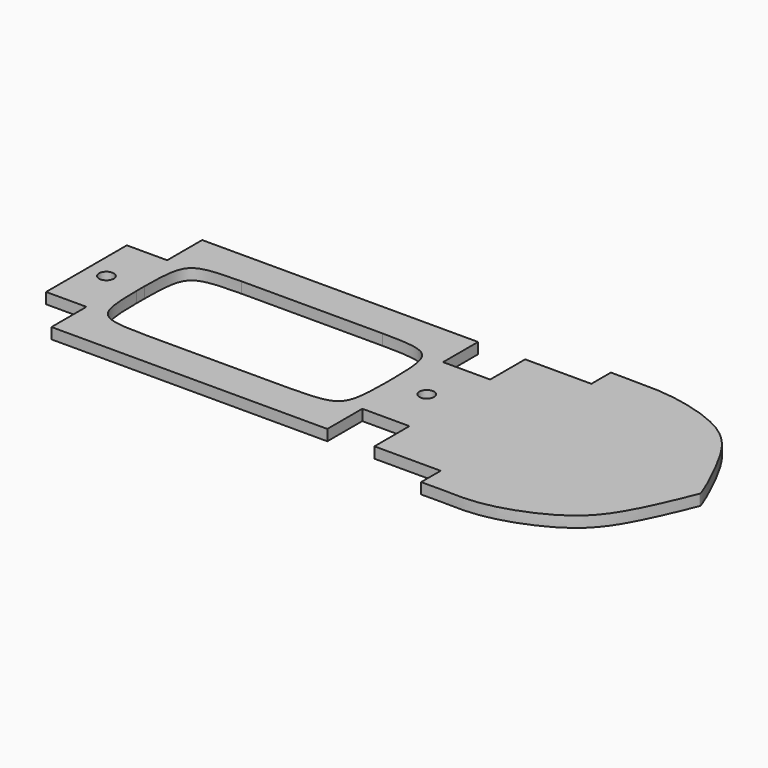
from build123d import *

# Parameters (mm, degrees)
F0_W        = 41.91
F0_H        = 19.05
F0_R        = 1.3890625
F0_W_2      = 52.07
F0_H_2      = 8.255
F0_W_3      = 7.62
F1_DEPTH    = 2.0574
F2_W        = 46.99
F2_H        = 22.225
F3_DEPTH    = 25.4
F4_T1_DEPTH = 2.0574
F6_DEPTH    = 2.0574


# Not quite as in the source:
# - a fillet or chamfer that OpenCascade refuses, or shapes differently, is made with other operations: its cross-section is extruded or revolved along the edge and cut away or added
# - a feature names something its author has since deleted; it is built from what else it names


with BuildPart() as f1:
    # F0 (on Top) → F1 (new body)
    with BuildSketch(Plane.XY):
        with Locations((29.845, 0)):
            Rectangle(F0_W, F0_H)
        with Locations((13.4267662017, 0)):
            Circle(F0_R, mode=Mode.SUBTRACT)
        with Locations((-17.145, -13.6525)):
            Rectangle(F0_W_2, F0_H_2)
        with Locations((-17.145, 0)):
            Rectangle(F0_W_2, F0_H)
        with Locations((-46.99, 0)):
            Rectangle(F0_W_3, F0_H)
        with Locations((-47.0252337983, 0)):
            Circle(F0_R, mode=Mode.SUBTRACT)
        with Locations((-17.145, 13.6525)):
            Rectangle(F0_W_2, F0_H_2)
    extrude(amount=F1_DEPTH)

    # F2 (on face) → F3 (cut)
    with BuildSketch(Plane.XY.offset(2.0574)):
        with Locations((-17.0991587498, 0)):
            Rectangle(F2_W, F2_H)
    extrude(amount=-F3_DEPTH, mode=Mode.SUBTRACT)

    # F4: fillet of radius 10.16 on 4 edges, made by hand

    # F4_s2 → F4_t1 (join)
    with BuildSketch(Plane.XY):
        with BuildLine():
            add(Edge.make_bspline(
                [(6.3958412502, 0.9525), (6.3958412502, 11.1125), (-3.7641587498, 11.1125)],
                knots=[0, 0, 0, 1, 1, 1], degree=2, weights=[1, 2.3333333333, 1]))
            Line((-3.7641587498, 11.1125), (6.3958412502, 11.1125))
            Line((6.3958412502, 11.1125), (6.3958412502, 0.9525))
        make_face()
        with BuildLine():
            add(Edge.make_bspline(
                [(-30.4341587498, 11.1125), (-40.5941587498, 11.1125), (-40.5941587498, 0.9525)],
                knots=[0, 0, 0, 1, 1, 1], degree=2, weights=[1, 2.3333333333, 1]))
            Line((-40.5941587498, 0.9525), (-40.5941587498, 11.1125))
            Line((-40.5941587498, 11.1125), (-30.4341587498, 11.1125))
        make_face()
        with BuildLine():
            add(Edge.make_bspline(
                [(-30.4341587498, -11.1125), (-40.5941587498, -11.1125), (-40.5941587498, -0.9525)],
                knots=[0, 0, 0, 1, 1, 1], degree=2, weights=[1, 2.3333333333, 1]))
            Line((-40.5941587498, -0.9525), (-40.5941587498, -11.1125))
            Line((-40.5941587498, -11.1125), (-30.4341587498, -11.1125))
        make_face()
        with BuildLine():
            add(Edge.make_bspline(
                [(-3.7641587498, -11.1125), (6.3958412502, -11.1125), (6.3958412502, -0.9525)],
                knots=[0, 0, 0, 1, 1, 1], degree=2, weights=[1, 2.3333333333, 1]))
            Line((6.3958412502, -0.9525), (6.3958412502, -11.1125))
            Line((6.3958412502, -11.1125), (-3.7641587498, -11.1125))
        make_face()
    extrude(amount=F4_T1_DEPTH)

    # F5 (on Top) → F6 (join)
    with BuildSketch(Plane.XY):
        with BuildLine():
            add(Edge.make_bspline(
                [(30.2796192753, 22.3951932201), (34.47761225, 22.2355197105), (40.54497388, 22.8560402759), (54.3807379627, 19.1979683007), (60.0879375817, 11.4498849698), (64.8467251166, 0.7216945038), (64.6662684157, 0.3740880638)],
                knots=[0, 0, 0, 0, 0.2383917442, 0.4983697633, 0.7405972723, 0.9754210457, 0.9754210457, 0.9754210457, 0.9754210457], degree=3))
            Line((30.2796192753, 22.3951932201), (30.2796192753, 17.78))
            Line((30.2796192753, 17.78), (17.78, 17.78))
            Line((17.78, 17.78), (17.78, 0))
            Line((17.78, 0), (17.78, -17.78))
            Line((17.78, -17.78), (30.2796192753, -17.78))
            Line((30.2796192753, -17.78), (30.2796192753, -22.3951932201))
            add(Edge.make_bspline(
                [(30.2796192753, -22.3951932201), (34.4859564493, -22.2352023333), (40.7613792543, -23.2344876139), (54.2509767666, -18.1718013245), (60.245134847, -10.8159221732), (64.5606245101, 0.1067004431), (64.6662684157, 0.3740880638)],
                knots=[0, 0, 0, 0, 0.2388655869, 0.4997646762, 0.7413186088, 0.9754893938, 0.9754893938, 0.9754893938, 0.9754893938], degree=3))
        make_face()
        with BuildLine():
            add(Edge.make_bspline(
                [(64.6662684157, 0.3740880638), (64.6773261408, 0.4020754691), (64.6662684157, 0.3740880638), (64.5520137623, 0.3740880638)],
                knots=[0.9754893938, 0.9754893938, 0.9754893938, 0.9754893938, 1, 1, 1, 1], degree=3))
            add(Edge.make_bspline(
                [(64.6662684157, 0.3740880638), (64.6473800513, 0.3377041719), (64.6008511396, 0.3553676853), (64.5520137623, 0.3740880638)],
                knots=[0.9754210457, 0.9754210457, 0.9754210457, 0.9754210457, 1, 1, 1, 1], degree=3))
        make_face(mode=Mode.SUBTRACT)
        with BuildLine():
            add(Edge.make_bspline(
                [(64.6662684157, 0.3740880638), (64.6473800513, 0.3377041719), (64.6008511396, 0.3553676853), (64.5520137623, 0.3740880638)],
                knots=[0.9754210457, 0.9754210457, 0.9754210457, 0.9754210457, 1, 1, 1, 1], degree=3))
            add(Edge.make_bspline(
                [(64.6662684157, 0.3740880638), (64.6773261408, 0.4020754691), (64.6662684157, 0.3740880638), (64.5520137623, 0.3740880638)],
                knots=[0.9754893938, 0.9754893938, 0.9754893938, 0.9754893938, 1, 1, 1, 1], degree=3))
        make_face()
    extrude(amount=F6_DEPTH)


solid = f1.part
